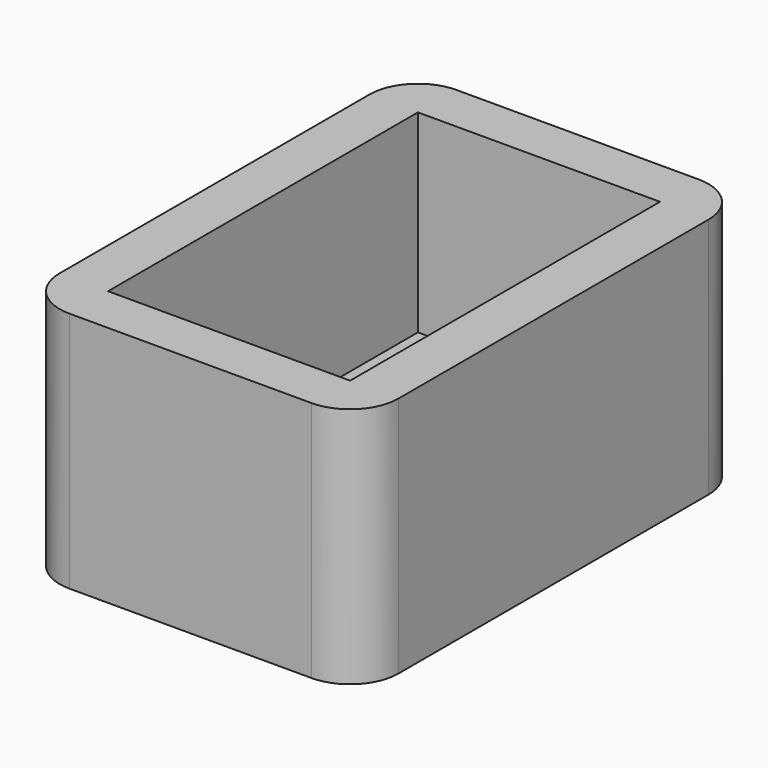
from build123d import *

# Parameters (mm, degrees)
F0_W     = 177.8
F0_H     = 127
F1_DEPTH = 254
F2_R     = 25.4
F3_T     = 25.4


# Not quite as in the source:
# - a shell that OpenCascade refuses in one call is made with other operations: the cavity is built on its own and cut out


with BuildPart() as f1:
    # F0 (on Front) → F1 (new body)
    with BuildSketch(Plane.XZ):
        with Locations((118.7249161303, 53.4633891671)):
            Rectangle(F0_W, F0_H)
    extrude(amount=-F1_DEPTH)

    # F2
    f2_edges = [f1.edges().sort_by_distance(p)[0] for p in [
        (207.624916, 0, 53.463389),
        (207.624916, 254, 53.463389),
        (29.824916, 254, 53.463389),
        (29.824916, 0, 53.463389),
    ]]
    fillet(f2_edges, radius=F2_R)

    # F3: shell of thickness 25.4, made by hand


with BuildPart() as f3_core1:
    # F3_t2: copy of F1
    add(f1.part)

    # the walls: a layer under each face that stays
    f3_faces = [f3_core1.faces().sort_by_distance(p)[0] for p in [
        (207.6249161303, 127, 53.4633891671),
        (118.7249161303, 0, 53.4633891671),
        (118.7249161303, 254, 53.4633891671),
        (29.8249161303, 127, 53.4633891671),
        (118.7249161303, 127, -10.0366108329),
    ]]
    thicken(f3_faces, amount=-F3_T, mode=Mode.SUBTRACT)


with BuildPart() as f1_1:
    add(f1.part)

    # what is left inside the walls is the cavity
    f3_cavity = [f3_core1.part.solids().sort_by_distance(p)[0] for p in [
        (118.724916, 160.866667, 15.617389),
    ]]
    add(f3_cavity, mode=Mode.SUBTRACT)


solid = f1_1.part
